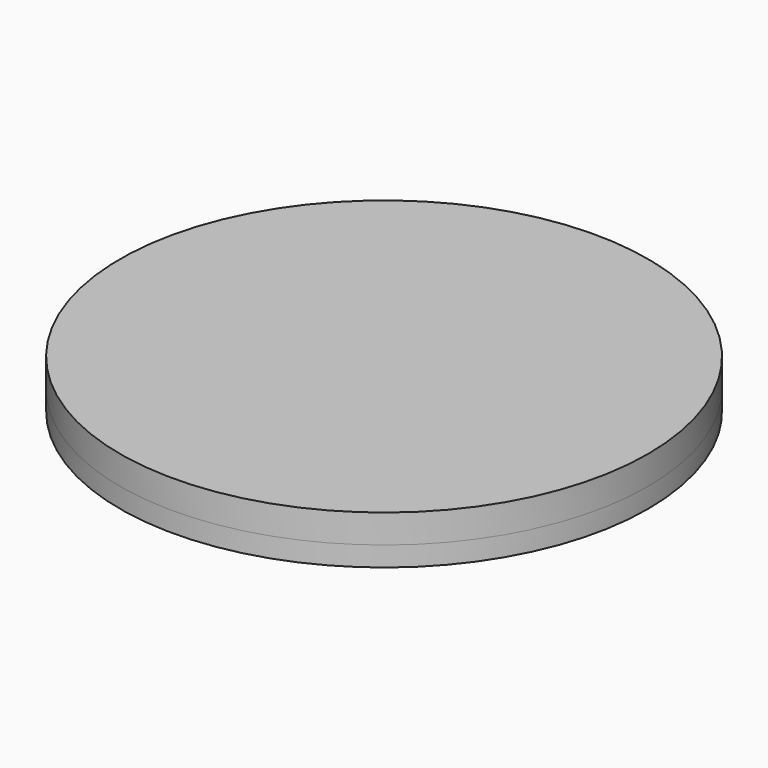
from build123d import *

# Parameters (mm, degrees)
F0_R     = 120
F0_R_2   = 100
F1_DEPTH = 9
F2_DEPTH = 4
F3_DEPTH = 13
F4_DEPTH = 9


with BuildPart() as f1:
    # F0 (on Top) → F1 (new body)
    with BuildSketch(Plane.XY):
        Circle(F0_R)
        Circle(F0_R_2, mode=Mode.SUBTRACT)
        Circle(F0_R_2)
    extrude(amount=-F1_DEPTH)

    # F0 (on Top) → F3 (join)
    with BuildSketch(Plane.XY):
        Circle(F0_R)
        Circle(F0_R_2, mode=Mode.SUBTRACT)
    extrude(amount=F3_DEPTH)



with BuildPart() as f2:
    # F0 (on Top) → F2 (new body)
    with BuildSketch(Plane.XY):
        Circle(F0_R_2)
    extrude(amount=F2_DEPTH)


with BuildPart() as f1_1:
    add(f1.part)
    # F4 (add): a face of the model
    f4_faces = [f2.part.faces().sort_by_distance(p)[0] for p in [
        (0, 0, 4),
    ]]
    extrude(f4_faces, amount=F4_DEPTH)


solid = Compound([f2.part, f1_1.part])
